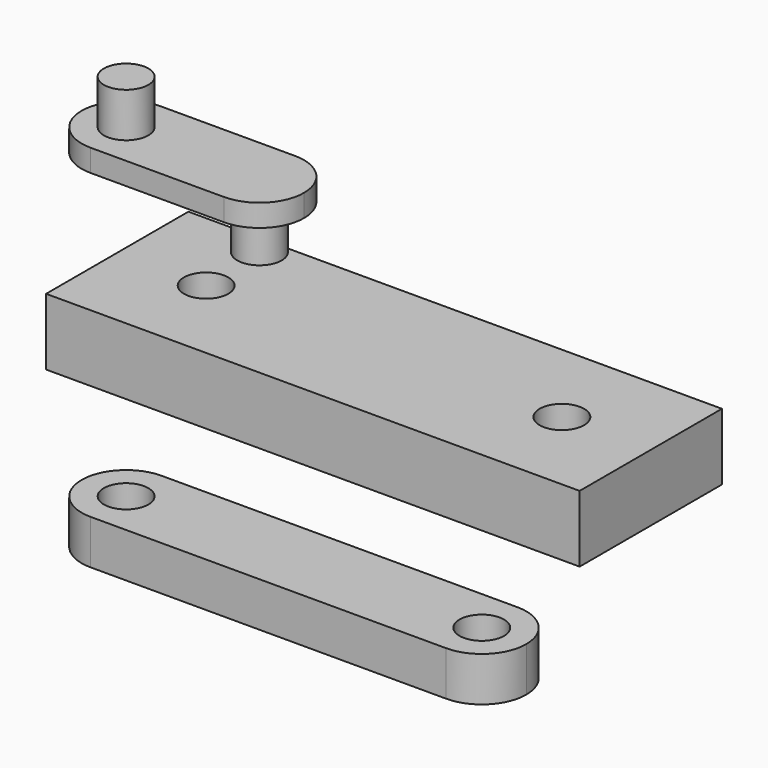
from build123d import *

# Parameters (mm, degrees)
F0_W      = 120
F0_H      = 15
F1_DEPTH  = 40
F2_R      = 5
F3_DEPTH  = 37.52124
F4_W      = 50
F4_H      = 5
F5_DEPTH  = 20
F8_DEPTH  = 10
F7_R      = 5
F9_DEPTH  = 10
F10_R     = 9.99999
F11_W     = 100
F11_H     = 10
F12_DEPTH = 20
F13_R     = 5
F14_DEPTH = 25
F15_R     = 9.99999


# Not quite as in the source:
# - a fillet or chamfer is up to 0.001 mm smaller than in the source, because OpenCascade refuses the exact size


with BuildPart() as f1:
    # F0 (on Front) → F1 (new body)
    with BuildSketch(Plane.XZ):
        with Locations((60, 7.5)):
            Rectangle(F0_W, F0_H)
    extrude(amount=-F1_DEPTH)

    # F2 (on face) → F3 (cut)
    with BuildSketch(Plane.XY.offset(15)):
        with Locations((20, 20)):
            Circle(F2_R)
        with Locations((100, 20)):
            Circle(F2_R)
    extrude(amount=-F3_DEPTH, mode=Mode.SUBTRACT)


with BuildPart() as f5:
    # F4 (on Front) → F5 (new body)
    with BuildSketch(Plane.XZ):
        with Locations((25, 44.6765302146)):
            Rectangle(F4_W, F4_H)
    extrude(amount=-F5_DEPTH)

    # F6 (on face) → F8 (join)
    with BuildSketch(Plane.XY.offset(47.1765302146)):
        with BuildLine():
            ThreePointArc((15, 10), (10, 15), (5, 10))
            ThreePointArc((5, 10), (10, 5), (15, 10))
        make_face()
    extrude(amount=F8_DEPTH)

    # F7 (on face) → F9 (join)
    with BuildSketch(Plane(origin=(0, 0, 42.1765302146), x_dir=(1, 0, 0), z_dir=(0, 0, -1))):
        with Locations((40, -10)):
            Circle(F7_R)
    extrude(amount=F9_DEPTH)

    # F10 (radius 10 in the source; OpenCascade refuses exactly that, so slightly less here)
    f10_edges = [f5.edges().sort_by_distance(p)[0] for p in [
        (0, 20, 44.67653),
        (0, 0, 44.67653),
        (50, 0, 44.67653),
        (50, 20, 44.67653),
    ]]
    fillet(f10_edges, radius=F10_R)


with BuildPart() as f12:
    # F11 (on Front) → F12 (new body)
    with BuildSketch(Plane.XZ):
        with Locations((50, -30.9100110515)):
            Rectangle(F11_W, F11_H)
    extrude(amount=-F12_DEPTH)

    # F13 (on face) → F14 (cut)
    with BuildSketch(Plane.XY.offset(-25.9100110515)):
        with BuildLine():
            ThreePointArc((5, 10), (10, 5), (15, 10))
            ThreePointArc((15, 10), (10, 15), (5, 10))
        make_face()
        with Locations((90, 10)):
            Circle(F13_R)
    extrude(amount=-F14_DEPTH, mode=Mode.SUBTRACT)

    # F15 (radius 10 in the source; OpenCascade refuses exactly that, so slightly less here)
    f15_edges = [f12.edges().sort_by_distance(p)[0] for p in [
        (0, 0, -30.910011),
        (0, 20, -30.910011),
        (100, 20, -30.910011),
        (100, 0, -30.910011),
    ]]
    fillet(f15_edges, radius=F15_R)


solid = Compound([f1.part, f5.part, f12.part])
